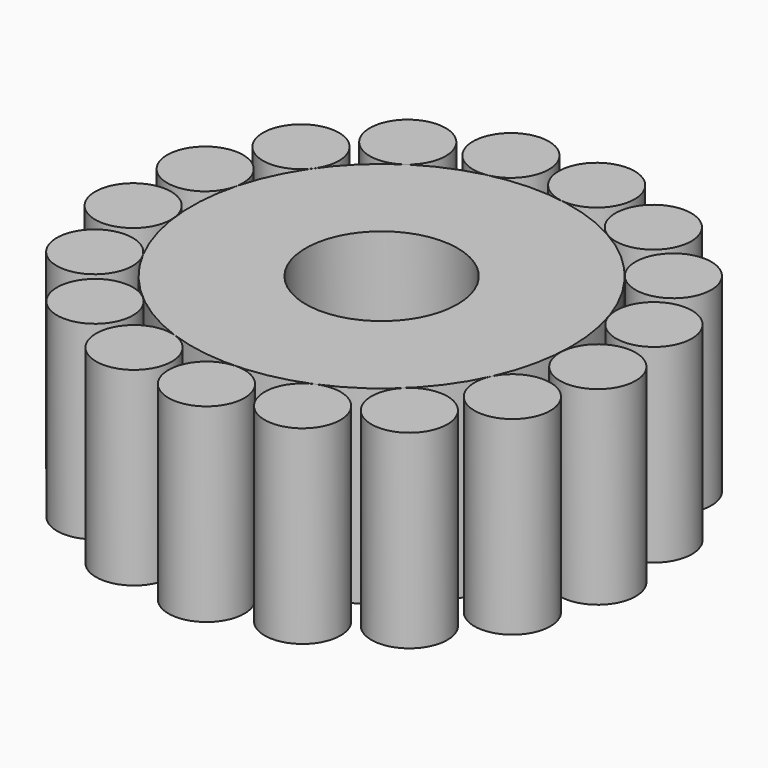
from build123d import *

# Parameters (mm, degrees)
F0_R     = 25
F1_DEPTH = 25
F2_R     = 10
F3_DEPTH = 25
F4_R     = 5
F5_DEPTH = 25
F6_COUNT = 17


with BuildPart() as f1:
    # F0 (on Top) → F1 (new body)
    with BuildSketch(Plane.XY):
        Circle(F0_R)
    extrude(amount=F1_DEPTH)

    # F2 (on face) → F3 (cut)
    with BuildSketch(Plane.XY.offset(25)):
        Circle(F2_R)
    extrude(amount=-F3_DEPTH, mode=Mode.SUBTRACT)


with BuildPart() as f5:
    # F4 (on Top) → F5 (new body)
    with BuildSketch(Plane.XY):
        with Locations((15, 25.9807621135)):
            Circle(F4_R)
    extrude(amount=F5_DEPTH)


with BuildPart() as f6_1:
    # F6: instance of F5
    add(f5.part.rotate(Axis((0, 0, 0), (0, 0, -1)), 1 * 360 / F6_COUNT))


with BuildPart() as f6_2:
    # F6: instance of F5
    add(f5.part.rotate(Axis((0, 0, 0), (0, 0, -1)), 2 * 360 / F6_COUNT))


with BuildPart() as f6_3:
    # F6: instance of F5
    add(f5.part.rotate(Axis((0, 0, 0), (0, 0, -1)), 3 * 360 / F6_COUNT))


with BuildPart() as f6_4:
    # F6: instance of F5
    add(f5.part.rotate(Axis((0, 0, 0), (0, 0, -1)), 4 * 360 / F6_COUNT))


with BuildPart() as f6_5:
    # F6: instance of F5
    add(f5.part.rotate(Axis((0, 0, 0), (0, 0, -1)), 5 * 360 / F6_COUNT))


with BuildPart() as f6_6:
    # F6: instance of F5
    add(f5.part.rotate(Axis((0, 0, 0), (0, 0, -1)), 6 * 360 / F6_COUNT))


with BuildPart() as f6_7:
    # F6: instance of F5
    add(f5.part.rotate(Axis((0, 0, 0), (0, 0, -1)), 7 * 360 / F6_COUNT))


with BuildPart() as f6_8:
    # F6: instance of F5
    add(f5.part.rotate(Axis((0, 0, 0), (0, 0, -1)), 8 * 360 / F6_COUNT))


with BuildPart() as f6_9:
    # F6: instance of F5
    add(f5.part.rotate(Axis((0, 0, 0), (0, 0, -1)), 9 * 360 / F6_COUNT))


with BuildPart() as f6_10:
    # F6: instance of F5
    add(f5.part.rotate(Axis((0, 0, 0), (0, 0, -1)), 10 * 360 / F6_COUNT))


with BuildPart() as f6_11:
    # F6: instance of F5
    add(f5.part.rotate(Axis((0, 0, 0), (0, 0, -1)), 11 * 360 / F6_COUNT))


with BuildPart() as f6_12:
    # F6: instance of F5
    add(f5.part.rotate(Axis((0, 0, 0), (0, 0, -1)), 12 * 360 / F6_COUNT))


with BuildPart() as f6_13:
    # F6: instance of F5
    add(f5.part.rotate(Axis((0, 0, 0), (0, 0, -1)), 13 * 360 / F6_COUNT))


with BuildPart() as f6_14:
    # F6: instance of F5
    add(f5.part.rotate(Axis((0, 0, 0), (0, 0, -1)), 14 * 360 / F6_COUNT))


with BuildPart() as f6_15:
    # F6: instance of F5
    add(f5.part.rotate(Axis((0, 0, 0), (0, 0, -1)), 15 * 360 / F6_COUNT))


with BuildPart() as f6_16:
    # F6: instance of F5
    add(f5.part.rotate(Axis((0, 0, 0), (0, 0, -1)), 16 * 360 / F6_COUNT))


solid = Compound([f1.part, f5.part, f6_1.part, f6_2.part, f6_3.part, f6_4.part, f6_5.part, f6_6.part, f6_7.part, f6_8.part, f6_9.part, f6_10.part, f6_11.part, f6_12.part, f6_13.part, f6_14.part, f6_15.part, f6_16.part])
